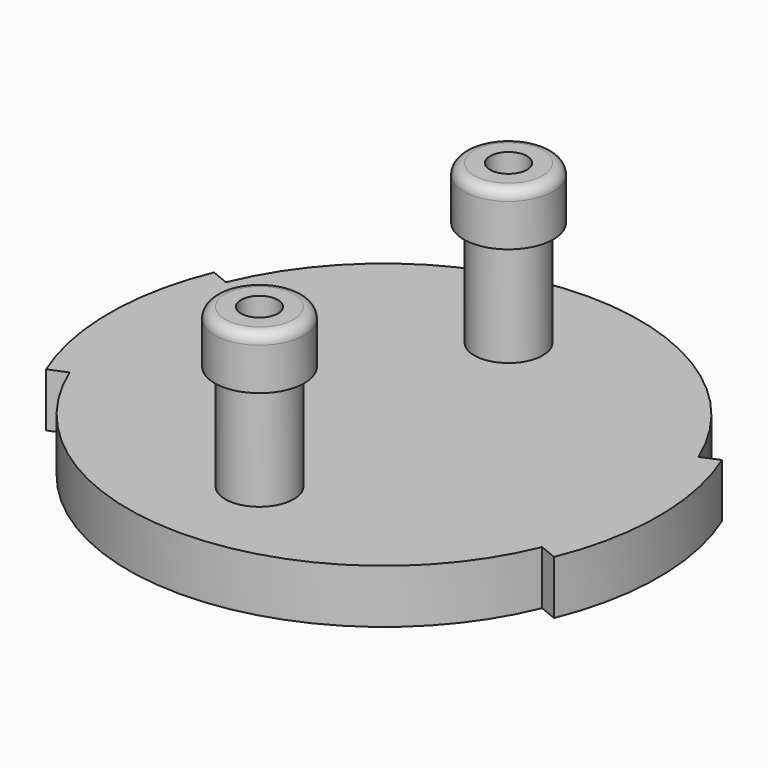
from build123d import *
from build123d import SkipClean  # not in build123d's __all__

# Parameters (mm, degrees)
F0_R      = 24.225
F1_DEPTH  = 5.1
F2_R      = 22.09
F2_R_2    = 21.09
F3_DEPTH  = 1
F5_DEPTH  = 1
F6_R      = 0.49999
F8_DEPTH  = 5.101
F9_R      = 3.25
F9_R_2    = 1.75
F10_DEPTH = 15
F12_DEPTH = 5.1
F14_R     = 4.25
F14_R_2   = 3.25
F15_DEPTH = 5
F16_R     = 0.99999


# Not quite as in the source:
# - a fillet or chamfer is up to 0.001 mm smaller than in the source, because OpenCascade refuses the exact size
# - after a boolean that leaves OpenCascade's solid faulty, fix() repairs it


with BuildPart() as f1:
    # F0 (on Top) → F1 (new body)
    with BuildSketch(Plane.XY):
        Circle(F0_R)
    extrude(amount=F1_DEPTH)

    # F2 (on face) → F3 (cut)
    with BuildSketch(Plane(origin=(0, 0, 0), x_dir=(1, 0, 0), z_dir=(0, 0, -1))):
        Circle(F2_R)
        Circle(F2_R_2, mode=Mode.SUBTRACT)
    extrude(amount=-F3_DEPTH, mode=Mode.SUBTRACT)

    # F4 (on face) → F5 (cut)
    with BuildSketch(Plane(origin=(0, 0, 0), x_dir=(1, 0, 0), z_dir=(0, 0, -1))):
        with BuildLine():
            Line((-12.0364031172, -15.25), (-1.6770509831, -15.25))
            ThreePointArc((-1.6770509831, -15.25), (1.75, -14.75), (-1.6770509831, -14.25))
            Line((-1.6770509831, -14.25), (-12.0364031172, -14.25))
            ThreePointArc((-12.0364031172, -14.25), (-13.4114031172, -12.875), (-12.0364031172, -11.5))
            Line((-12.0364031172, -11.5), (15.5643824163, -11.5))
            ThreePointArc((15.5643824163, -11.5), (17.0643824163, -10), (15.5643824163, -8.5))
            Line((15.5643824163, -8.5), (-16.6808273176, -8.5))
            ThreePointArc((-16.6808273176, -8.5), (-17.1808273176, -8), (-16.6808273176, -7.5))
            Line((-16.6808273176, -7.5), (17.5, -7.5))
            ThreePointArc((17.5, -7.5), (19, -6), (17.5, -4.5))
            Line((17.5, -4.5), (-18.0623918682, -4.5))
            ThreePointArc((-18.0623918682, -4.5), (-18.5623918682, -4), (-18.0623918682, -3.5))
            Line((-18.0623918682, -3.5), (18.3915741577, -3.5))
            ThreePointArc((18.3915741577, -3.5), (19.8915741577, -2), (18.3915741577, -0.5))
            Line((18.3915741577, -0.5), (-18.5, -0.5))
            ThreePointArc((-18.5, -0.5), (-19, 0), (-18.5, 0.5))
            Line((-18.5, 0.5), (18.3915741577, 0.5))
            ThreePointArc((18.3915741577, 0.5), (19.8915741577, 2), (18.3915741577, 3.5))
            Line((18.3915741577, 3.5), (-18.0623918682, 3.5))
            ThreePointArc((-18.0623918682, 3.5), (-18.5623918682, 4), (-18.0623918682, 4.5))
            Line((-18.0623918682, 4.5), (17.5, 4.5))
            ThreePointArc((17.5, 4.5), (19, 6), (17.5, 7.5))
            Line((17.5, 7.5), (-16.6808273176, 7.5))
            ThreePointArc((-16.6808273176, 7.5), (-17.1808273176, 8), (-16.6808273176, 8.5))
            Line((-16.6808273176, 8.5), (15.5643824163, 8.5))
            ThreePointArc((15.5643824163, 8.5), (17.0643824163, 10), (15.5643824163, 11.5))
            Line((15.5643824163, 11.5), (-12.0364031172, 11.5))
            ThreePointArc((-12.0364031172, 11.5), (-13.4114031172, 12.875), (-12.0364031172, 14.25))
            Line((-12.0364031172, 14.25), (-1.6770509831, 14.25))
            ThreePointArc((-1.6770509831, 14.25), (1.75, 14.75), (-1.6770509831, 15.25))
            Line((-1.6770509831, 15.25), (-12.0364031172, 15.25))
            ThreePointArc((-12.0364031172, 15.25), (-14.4114031172, 12.875), (-12.0364031172, 10.5))
            Line((-12.0364031172, 10.5), (15.5643824163, 10.5))
            ThreePointArc((15.5643824163, 10.5), (16.0643824163, 10), (15.5643824163, 9.5))
            Line((15.5643824163, 9.5), (-16.6808273176, 9.5))
            ThreePointArc((-16.6808273176, 9.5), (-18.1808273176, 8), (-16.6808273176, 6.5))
            Line((-16.6808273176, 6.5), (17.5, 6.5))
            ThreePointArc((17.5, 6.5), (18, 6), (17.5, 5.5))
            Line((17.5, 5.5), (-18.0623918682, 5.5))
            ThreePointArc((-18.0623918682, 5.5), (-19.5623918682, 4), (-18.0623918682, 2.5))
            Line((-18.0623918682, 2.5), (18.3915741577, 2.5))
            ThreePointArc((18.3915741577, 2.5), (18.8915741577, 2), (18.3915741577, 1.5))
            Line((18.3915741577, 1.5), (-18.5, 1.5))
            ThreePointArc((-18.5, 1.5), (-20, 0), (-18.5, -1.5))
            Line((-18.5, -1.5), (18.3915741577, -1.5))
            ThreePointArc((18.3915741577, -1.5), (18.8915741577, -2), (18.3915741577, -2.5))
            Line((18.3915741577, -2.5), (-18.0623918682, -2.5))
            ThreePointArc((-18.0623918682, -2.5), (-19.5623918682, -4), (-18.0623918682, -5.5))
            Line((-18.0623918682, -5.5), (17.5, -5.5))
            ThreePointArc((17.5, -5.5), (18, -6), (17.5, -6.5))
            Line((17.5, -6.5), (-16.6808273176, -6.5))
            ThreePointArc((-16.6808273176, -6.5), (-18.1808273176, -8), (-16.6808273176, -9.5))
            Line((-16.6808273176, -9.5), (15.5643824163, -9.5))
            ThreePointArc((15.5643824163, -9.5), (16.0643824163, -10), (15.5643824163, -10.5))
            Line((15.5643824163, -10.5), (-12.0364031172, -10.5))
            ThreePointArc((-12.0364031172, -10.5), (-14.4114031172, -12.875), (-12.0364031172, -15.25))
        make_face()
    extrude(amount=-F5_DEPTH, mode=Mode.SUBTRACT)

    # F6 (radius 0.5 in the source; OpenCascade refuses exactly that, so slightly less here)
    f6_edges = [f1.edges().sort_by_distance(p)[0] for p in [
        (16.064382, 10, 1),
        (1.76399, 10.5, 1),
        (-14.411403, 12.875, 1),
        (-6.856727, 15.25, 1),
        (1.75, 14.75, 1),
        (-6.856727, 14.25, 1),
        (-13.411403, 12.875, 1),
        (1.76399, 11.5, 1),
        (17.064382, 10, 1),
        (-0.558222, 8.5, 1),
        (-17.180827, 8, 1),
        (0.409586, 7.5, 1),
        (19, 6, 1),
        (-0.281196, 4.5, 1),
        (-18.562392, 4, 1),
        (0.164591, 3.5, 1),
        (19.891574, 2, 1),
        (-0.054213, 0.5, 1),
        (-19, 0, 1),
        (-0.054213, -0.5, 1),
        (19.891574, -2, 1),
        (0.164591, -3.5, 1),
        (-18.562392, -4, 1),
        (-0.281196, -4.5, 1),
        (19, -6, 1),
        (0.409586, -7.5, 1),
        (-17.180827, -8, 1),
        (-0.558222, -8.5, 1),
        (17.064382, -10, 1),
        (1.76399, -11.5, 1),
        (-13.411403, -12.875, 1),
        (-6.856727, -14.25, 1),
        (1.75, -14.75, 1),
        (-6.856727, -15.25, 1),
        (-14.411403, -12.875, 1),
        (1.76399, -10.5, 1),
        (16.064382, -10, 1),
        (-0.558222, -9.5, 1),
        (-18.180827, -8, 1),
        (0.409586, -6.5, 1),
        (18, -6, 1),
        (-0.281196, -5.5, 1),
        (-19.562392, -4, 1),
        (0.164591, -2.5, 1),
        (18.891574, -2, 1),
        (-0.054213, -1.5, 1),
        (-20, 0, 1),
        (-0.054213, 1.5, 1),
        (18.891574, 2, 1),
        (0.164591, 2.5, 1),
        (-19.562392, 4, 1),
        (-0.281196, 5.5, 1),
        (18, 6, 1),
        (0.409586, 6.5, 1),
        (-18.180827, 8, 1),
        (-0.558222, 9.5, 1),
    ]]
    fillet(f6_edges, radius=F6_R)

    # F7 (on face) → F8 (cut, through all)
    with BuildSketch(Plane(origin=(0, 0, 0), x_dir=(1, 0, 0), z_dir=(0, 0, -1))):
        with BuildLine():
            ThreePointArc((-1.6770509831, 14.25), (1.75, 14.75), (-1.6770509831, 15.25))
            ThreePointArc((-1.6770509831, 15.25), (-1.75, 14.75), (-1.6770509831, 14.25))
        make_face()
        with BuildLine():
            ThreePointArc((-1.6770509831, -14.25), (-1.75, -14.75), (-1.6770509831, -15.25))
            ThreePointArc((-1.6770509831, -15.25), (1.75, -14.75), (-1.6770509831, -14.25))
        make_face()
    extrude(amount=-F8_DEPTH, mode=Mode.SUBTRACT)

    # F9 (on face) → F10 (join)
    with BuildSketch(Plane.XY.offset(5.1)):
        with Locations((0, 14.75)):
            Circle(F9_R)
        with Locations((0, 14.75)):
            Circle(F9_R_2, mode=Mode.SUBTRACT)
        with Locations((0, -14.75)):
            Circle(F9_R)
        with Locations((0, -14.75)):
            Circle(F9_R_2, mode=Mode.SUBTRACT)
    with SkipClean():  # cleaning this boolean's faces spoils the solid; the shape is the same uncleaned
        extrude(amount=F10_DEPTH)

    # F11 (on Top) → F12 (join, through all)
    with BuildSketch(Plane.XY):
        with BuildLine():
            Line((-22.3858222692, 9.2588112807), (-24.060719025, 9.945))
            ThreePointArc((-24.060719025, 9.945), (-26.035, 0), (-24.060719025, -9.945))
            Line((-24.060719025, -9.945), (-22.3879745873, -9.2536057231))
            ThreePointArc((-22.3879745873, -9.2536057231), (-24.2249998363, 0.0028164829), (-22.3858222692, 9.2588112807))
        make_face()
        with BuildLine():
            Line((22.3879745873, -9.2536057231), (24.060719025, -9.945))
            ThreePointArc((24.060719025, -9.945), (26.035, 0), (24.060719025, 9.945))
            Line((24.060719025, 9.945), (22.3879745873, 9.2536057231))
            ThreePointArc((22.3879745873, 9.2536057231), (24.225, 0), (22.3879745873, -9.2536057231))
        make_face()
    extrude(amount=F12_DEPTH)

    add(f1.part.fix(), mode=Mode.REPLACE)

    # F14 (on offset) → F15 (join, through all)
    with BuildSketch(Plane.XY.offset(15.1)):
        with Locations((0, 14.75)):
            Circle(F14_R)
        with Locations((0, 14.75)):
            Circle(F14_R_2, mode=Mode.SUBTRACT)
        with Locations((0, -14.75)):
            Circle(F14_R)
        with Locations((0, -14.75)):
            Circle(F14_R_2, mode=Mode.SUBTRACT)
    extrude(amount=F15_DEPTH)

    # F16 (radius 1 in the source; OpenCascade refuses exactly that, so slightly less here)
    f16_edges = [f1.edges().sort_by_distance(p)[0] for p in [
        (-4.25, 14.75, 20.1),
        (-4.25, -14.75, 20.1),
    ]]
    fillet(f16_edges, radius=F16_R)


solid = f1.part
